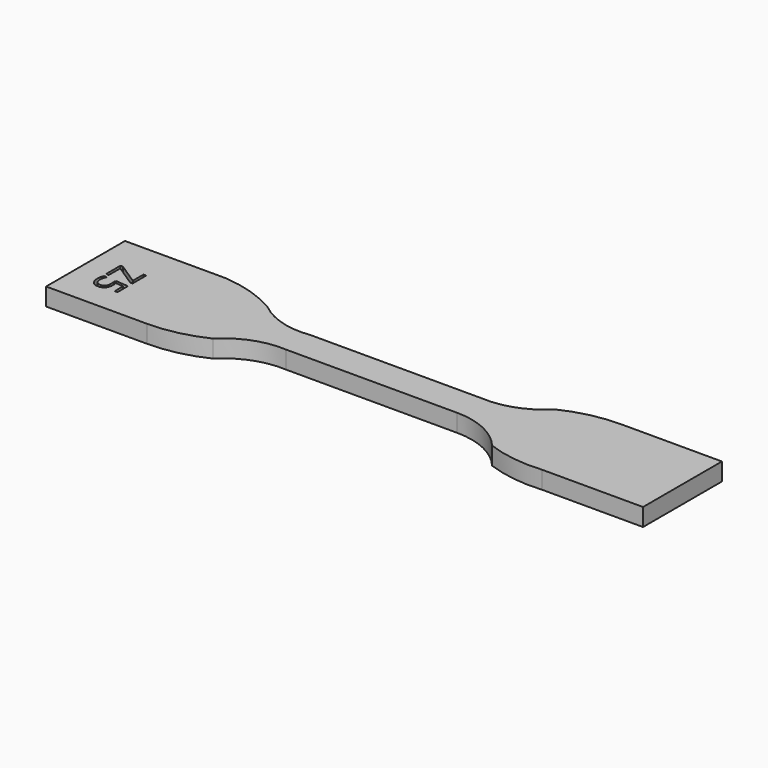
from build123d import *

# Parameters (mm, degrees)
F1_DEPTH     = 3.4
F2_TEXT_SIZE = 7.0564552314
F3_DEPTH     = 1


# Not quite as in the source:
# - Text() gives the source's letters only with a copy of the font that has no kerning and outlines rounded to 1/6400 em; it was checked with that copy


with BuildPart() as f1:
    # F0 (on Top) → F1 (new body)
    with BuildSketch(Plane.XY):
        with BuildLine():
            Line((-14.4320548165, 19.7811394548), (-33.8720548165, 19.7811394548))
            Line((-33.8720548165, 19.7811394548), (-33.8720548165, 0.7811394548))
            Line((-33.8720548165, 0.7811394548), (-14.4320548165, 0.7811394548))
            ThreePointArc((-14.4320548165, 0.7811394548), (-8.9053122052, 1.3996892086), (-3.6520548165, 3.2247301661))
            ThreePointArc((-3.6520548165, 3.2247301661), (1.3014698263, 6.4128780055), (7.1279451835, 7.2811394548))
            Line((7.1279451835, 7.2811394548), (40.1279451835, 7.2811394548))
            ThreePointArc((40.1279451835, 7.2811394548), (46.0837574042, 5.9511158081), (50.9079451835, 2.2137538538))
            ThreePointArc((50.9079451835, 2.2137538538), (56.2191047011, 0.9041953221), (61.6879451835, 0.7811394548))
            Line((61.6879451835, 0.7811394548), (81.1279451835, 0.7811394548))
            Line((81.1279451835, 0.7811394548), (81.1279451835, 19.7811394548))
            Line((81.1279451835, 19.7811394548), (61.6879451835, 19.7811394548))
            ThreePointArc((61.6879451835, 19.7811394548), (56.1612025723, 19.162589701), (50.9079451835, 17.3375487435))
            ThreePointArc((50.9079451835, 17.3375487435), (45.9544205407, 14.1494009041), (40.1279451835, 13.2811394548))
            Line((40.1279451835, 13.2811394548), (7.1279451835, 13.2811394548))
            ThreePointArc((7.1279451835, 13.2811394548), (1.4167452884, 13.6925537245), (-3.6520548165, 16.3560723447))
            ThreePointArc((-3.6520548165, 16.3560723447), (-8.8458057958, 18.686276846), (-14.4320548165, 19.7811394548))
        make_face()
    extrude(amount=F1_DEPTH)

    # F2 (on face) → F3 (cut)
    with BuildSketch(Plane.XY.offset(3.4)):
        with Locations(Location((-29.3720550835, 13.353464842), (0, 0, -90))):
            Text('Z5', F2_TEXT_SIZE, font='Open Sans', text_align=(TextAlign.LEFT, TextAlign.BOTTOM))
    extrude(amount=-F3_DEPTH, mode=Mode.SUBTRACT)


solid = f1.part
